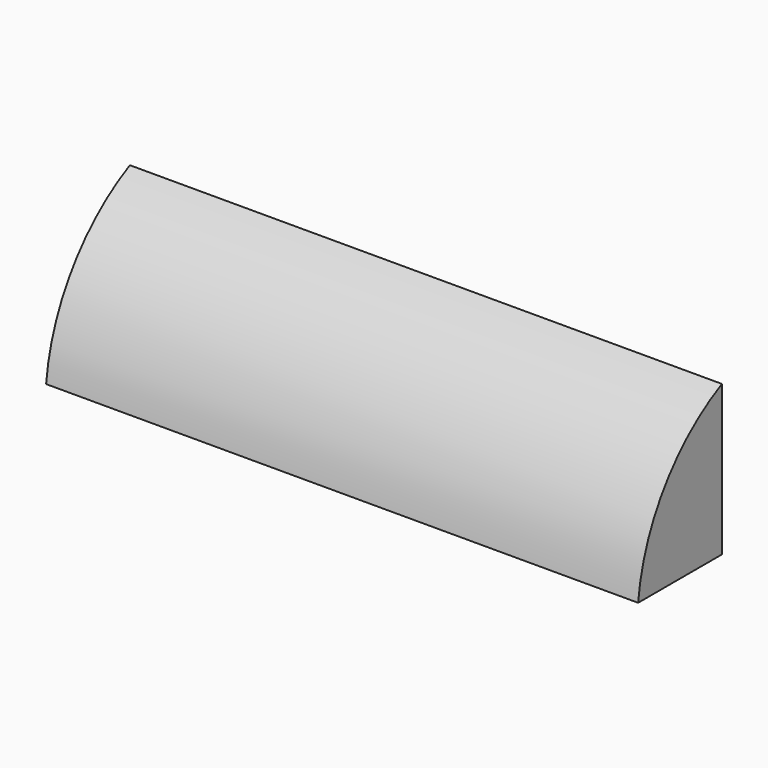
from build123d import *

# Parameters (mm, degrees)
F0_W        = 7.112
F0_H        = 1.8034
F1_DEPTH    = 1.27
F2_W        = 6.0393624008
F2_H        = 0.5219200684
F3_DEPTH    = 0.6604
F4_T1_DEPTH = 17.2978356076


# Not quite as in the source:
# - a fillet or chamfer that OpenCascade refuses, or shapes differently, is made with other operations: its cross-section is extruded or revolved along the edge and cut away or added


with BuildPart() as f1:
    # F0 (on Front) → F1 (new body)
    with BuildSketch(Plane.XZ):
        with Locations((-54.2522707031, 39.2414294181)):
            Rectangle(F0_W, F0_H)
    extrude(amount=F1_DEPTH)

    # F2 (on face) → F3 (cut)
    with BuildSketch(Plane(origin=(0, 0, 38.3397294181), x_dir=(1, 0, 0), z_dir=(0, 0, -1))):
        with Locations((-54.2349088937, 0.599740466)):
            Rectangle(F2_W, F2_H)
    extrude(amount=-F3_DEPTH, mode=Mode.SUBTRACT)

    # F4: fillet of radius 2.2688779059 on 1 edges, made by hand

    # F4_s2 → F4_t1 (cut)
    with BuildSketch(Plane.YZ.offset(-62.9011885069)):
        with BuildLine():
            ThreePointArc((0, 40.1431294181), (-0.9264972476, 39.3062695365), (-1.27, 38.1059622966))
            Line((-1.27, 38.1059622966), (-1.27, 40.1431294181))
            Line((-1.27, 40.1431294181), (0, 40.1431294181))
        make_face()
    extrude(amount=F4_T1_DEPTH, mode=Mode.SUBTRACT)


solid = f1.part
